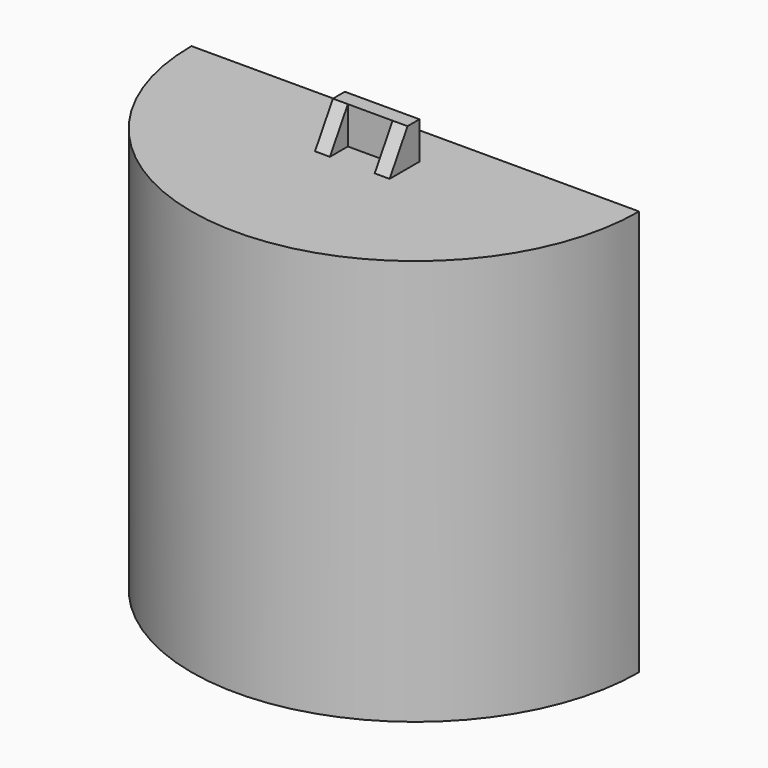
from build123d import *

# Parameters (mm, degrees)
F1_DEPTH       = 4.7625
F3_DEPTH       = 127
F5_DEPTH       = 6.35
F7_DEPTH       = 12.7
F9_DEPTH       = 5.08
F11_ANGLE_BACK = 20
F11_ANGLE      = 40
F12_R          = 5.08


# Not quite as in the source:
# - a length typed as a fraction of an inch, garbled in the dataset ("3 / 203.2 mm" for 3/8 in), is restored
# - a pattern or mirror of a feature is missing from the dataset's text; its kind, count and spacing are read off the source's solid


with BuildPart() as f1:
    # F0 (on Top) → F1 (new body)
    with BuildSketch(Plane.XY):
        with BuildLine():
            ThreePointArc((-76.2, 0), (0, -76.2), (76.2, 0))
            Line((76.2, 0), (67.31, 0))
            Line((67.31, 0), (67.31, -12.7))
            Line((67.31, -12.7), (-67.31, -12.7))
            Line((-67.31, -12.7), (-67.31, 0))
            Line((-67.31, 0), (-76.2, 0))
        make_face()
    extrude(amount=F1_DEPTH)

    # F2 (on face) → F3 (join)
    with BuildSketch(Plane.XY.offset(4.7625)):
        with BuildLine():
            Line((-67.31, 0), (-76.2, 0))
            ThreePointArc((-76.2, 0), (0, -76.2), (76.2, 0))
            Line((76.2, 0), (67.31, 0))
            ThreePointArc((67.31, 0), (0, -67.31), (-67.31, 0))
        make_face()
    extrude(amount=F3_DEPTH)

    # F4 (on face) → F5 (join)
    with BuildSketch(Plane.XY.offset(131.7625)):
        with BuildLine():
            Line((76.2, 0), (-76.2, 0))
            ThreePointArc((-76.2, 0), (0, -76.2), (76.2, 0))
        make_face()
    extrude(amount=F5_DEPTH)

    # F6 (on face) → F7 (join)
    with BuildSketch(Plane.XY.offset(138.1125)):
        Polygon((12.7, -14.0898204726), (0, -14.0898204726), (-12.7, -14.0898204726), (-12.7, -19.1698204726), (0, -19.1698204726), (12.7, -19.1698204726), align=None)
    extrude(amount=F7_DEPTH)

    # F8 (on face) → F9 (join)
    with BuildSketch(Plane.YZ.offset(12.7)):
        Polygon((-19.1698204726, 150.8125), (-26.7898204726, 138.1125), (-19.1698204726, 138.1125), align=None)
    f9 = extrude(amount=-F9_DEPTH)

    # F9_copies: F9 across plane
    add(f9.mirror(Plane(origin=(0, 0, 0), x_dir=(0, 0, -1), z_dir=(-1, 0, 0))))


with BuildPart() as f11:
    # F10 (on Right) → F11 (revolve)
    with BuildSketch(Plane.YZ, mode=Mode.PRIVATE) as f11_sk:
        Polygon((-98.6883191255, -24.4902079291), (-69.5020258427, 0), (-76.2, 0), (-76.2, 5.1620067097), (-104.2903103798, -17.814014726), align=None)
    revolve(f11_sk.sketch.rotate(Axis((0, 0, 0), (0, 0, -1)), -F11_ANGLE_BACK), axis=Axis((0, 0, 0), (0, 0, -1)), revolution_arc=F11_ANGLE)

    # F12
    f12_edges = [f11.edges().sort_by_distance(p)[0] for p in [
        (34.71139, -95.36876, -21.152111),
        (-34.71139, -95.36876, -21.152111),
    ]]
    fillet(f12_edges, radius=F12_R)


solid = f1.part
